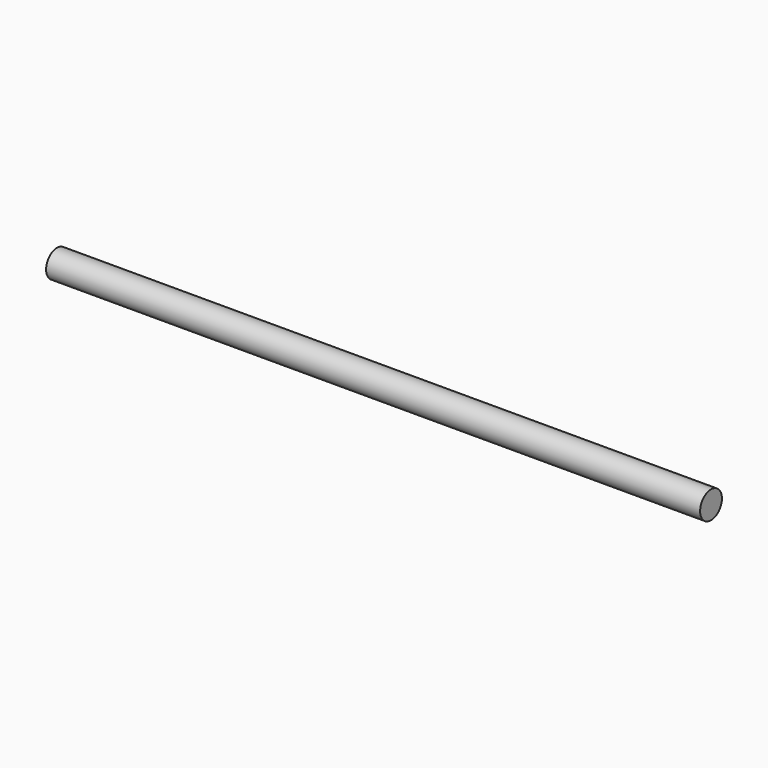
from build123d import *


# Not quite as in the source:
# - the program builds the solid bodies; features that only make, move or delete a surface that nothing else refers to are left out


with BuildPart() as f2:
    # F0 (on Front) → F2 (revolve)
    with BuildSketch(Plane.XZ):
        Polygon((-457.2, -175.1871720561), (-457.2, -194.2371720561), (457.2, -194.2371720561), (457.2, -175.1871720561), (0, -175.1871720561), align=None)
    revolve(axis=Axis((0, 0, -194.2371720561), (1, 0, 0)))


solid = f2.part
